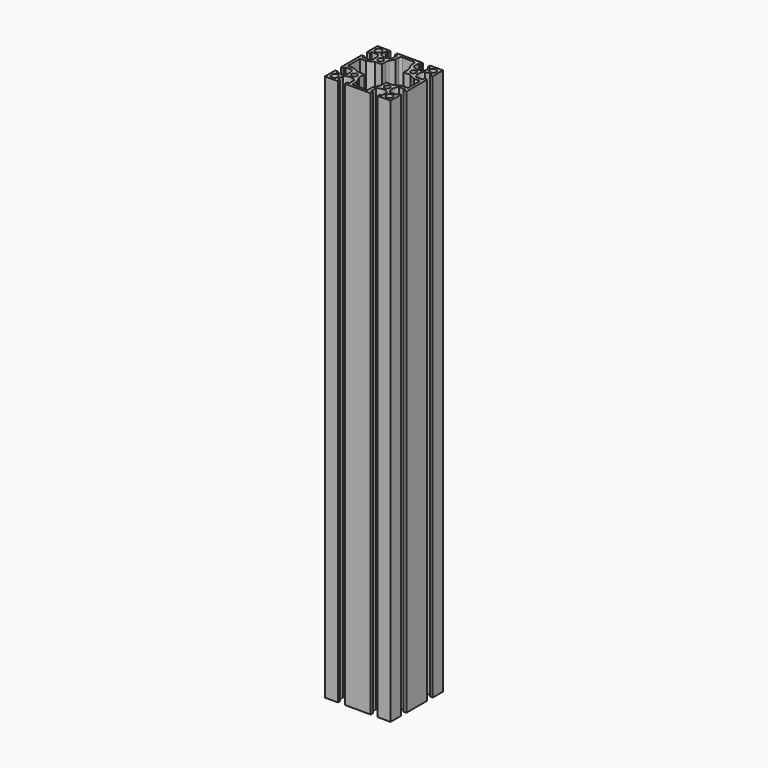
from build123d import *

# Parameters (mm, degrees)
F0_R     = 3
F0_R_2   = 2.5
F1_DEPTH = 500
F2_R     = 2
F3_R     = 7


# Not quite as in the source:
# - a feature names something its author has since deleted; it is built from what else it names


with BuildPart() as f1:
    # F0 (on Top) → F1 (new body)
    with BuildSketch(Plane.XY):
        with BuildLine():
            Line((18.15, -30), (30, -30))
            Line((30, -30), (30, -18.15))
            Line((30, -18.15), (27.5, -18.15))
            Line((27.5, -18.15), (27.5, -20.15))
            Line((27.5, -20.15), (21.5477069044, -20.15))
            ThreePointArc((21.5477069044, -20.15), (19.5, -15), (21.5477069044, -9.85))
            Line((21.5477069044, -9.85), (27.5, -9.85))
            Line((27.5, -9.85), (27.5, -11.85))
            Line((27.5, -11.85), (30, -11.85))
            Line((30, -11.85), (30, 11.85))
            Line((30, 11.85), (27.5, 11.85))
            Line((27.5, 11.85), (27.5, 9.85))
            Line((27.5, 9.85), (21.5477069044, 9.85))
            ThreePointArc((21.5477069044, 9.85), (19.5, 15), (21.5477069044, 20.15))
            Line((21.5477069044, 20.15), (27.5, 20.15))
            Line((27.5, 20.15), (27.5, 18.15))
            Line((27.5, 18.15), (30, 18.15))
            Line((30, 18.15), (30, 30))
            Line((30, 30), (18.15, 30))
            Line((18.15, 30), (18.15, 27.5))
            Line((18.15, 27.5), (20.15, 27.5))
            Line((20.15, 27.5), (20.15, 21.5477069044))
            ThreePointArc((20.15, 21.5477069044), (15, 19.5), (9.85, 21.5477069044))
            Line((9.85, 21.5477069044), (9.85, 27.5))
            Line((9.85, 27.5), (11.85, 27.5))
            Line((11.85, 27.5), (11.85, 30))
            Line((11.85, 30), (-11.85, 30))
            Line((-11.85, 30), (-11.85, 27.5))
            Line((-11.85, 27.5), (-9.85, 27.5))
            Line((-9.85, 27.5), (-9.85, 21.5477069044))
            ThreePointArc((-9.85, 21.5477069044), (-15, 19.5), (-20.15, 21.5477069044))
            Line((-20.15, 21.5477069044), (-20.15, 27.5))
            Line((-20.15, 27.5), (-18.15, 27.5))
            Line((-18.15, 27.5), (-18.15, 30))
            Line((-18.15, 30), (-30, 30))
            Line((-30, 30), (-30, 18.15))
            Line((-30, 18.15), (-27.5, 18.15))
            Line((-27.5, 18.15), (-27.5, 20.15))
            Line((-27.5, 20.15), (-21.5477069044, 20.15))
            ThreePointArc((-21.5477069044, 20.15), (-19.5, 15), (-21.5477069044, 9.85))
            Line((-21.5477069044, 9.85), (-27.5, 9.85))
            Line((-27.5, 9.85), (-27.5, 11.85))
            Line((-27.5, 11.85), (-30, 11.85))
            Line((-30, 11.85), (-30, -11.85))
            Line((-30, -11.85), (-27.5, -11.85))
            Line((-27.5, -11.85), (-27.5, -9.85))
            Line((-27.5, -9.85), (-21.5477069044, -9.85))
            ThreePointArc((-21.5477069044, -9.85), (-19.5, -15), (-21.5477069044, -20.15))
            Line((-21.5477069044, -20.15), (-27.5, -20.15))
            Line((-27.5, -20.15), (-27.5, -18.15))
            Line((-27.5, -18.15), (-30, -18.15))
            Line((-30, -18.15), (-30, -30))
            Line((-30, -30), (-18.15, -30))
            Line((-18.15, -30), (-18.15, -27.5))
            Line((-18.15, -27.5), (-20.15, -27.5))
            Line((-20.15, -27.5), (-20.15, -21.5477069044))
            ThreePointArc((-20.15, -21.5477069044), (-15, -19.5), (-9.85, -21.5477069044))
            Line((-9.85, -21.5477069044), (-9.85, -27.5))
            Line((-9.85, -27.5), (-11.85, -27.5))
            Line((-11.85, -27.5), (-11.85, -30))
            Line((-11.85, -30), (11.85, -30))
            Line((11.85, -30), (11.85, -27.5))
            Line((11.85, -27.5), (9.85, -27.5))
            Line((9.85, -27.5), (9.85, -21.5477069044))
            ThreePointArc((9.85, -21.5477069044), (15, -19.5), (20.15, -21.5477069044))
            Line((20.15, -21.5477069044), (20.15, -27.5))
            Line((20.15, -27.5), (18.15, -27.5))
            Line((18.15, -27.5), (18.15, -30))
        make_face()
        with Locations((-25, -25)):
            Circle(F0_R, mode=Mode.SUBTRACT)
        with Locations((-15, -15)):
            Circle(F0_R_2, mode=Mode.SUBTRACT)
        with Locations((25, -25)):
            Circle(F0_R, mode=Mode.SUBTRACT)
        with Locations((15, -15)):
            Circle(F0_R_2, mode=Mode.SUBTRACT)
        with Locations((-25, 25)):
            Circle(F0_R, mode=Mode.SUBTRACT)
        with Locations((-15, 15)):
            Circle(F0_R_2, mode=Mode.SUBTRACT)
        Polygon((-7, 22), (-7, 27.5), (0, 27.5), (7, 27.5), (7, 22), (10, 16), (10, 10), (16, 10), (22, 7), (27.5, 7), (27.5, 0), (27.5, -7), (22, -7), (16, -10), (10, -10), (10, -16), (7, -22), (7, -27.5), (0, -27.5), (-7, -27.5), (-7, -22), (-10, -16), (-10, -10), (-16, -10), (-22, -7), (-27.5, -7), (-27.5, 0), (-27.5, 7), (-22, 7), (-16, 10), (-10, 10), (-10, 16), align=None, mode=Mode.SUBTRACT)
        with Locations((15, 15)):
            Circle(F0_R_2, mode=Mode.SUBTRACT)
        with Locations((25, 25)):
            Circle(F0_R, mode=Mode.SUBTRACT)
    extrude(amount=F1_DEPTH)

    # F2
    f2_edges = [f1.edges().sort_by_distance(p)[0] for p in [
        (-7, 27.5, 250),
        (7, 27.5, 250),
    ]]
    fillet(f2_edges, radius=F2_R)

    # F3
    f3_edges = [f1.edges().sort_by_distance(p)[0] for p in [
        (-10, 16, 250),
        (10, 16, 250),
    ]]
    fillet(f3_edges, radius=F3_R)


solid = f1.part
